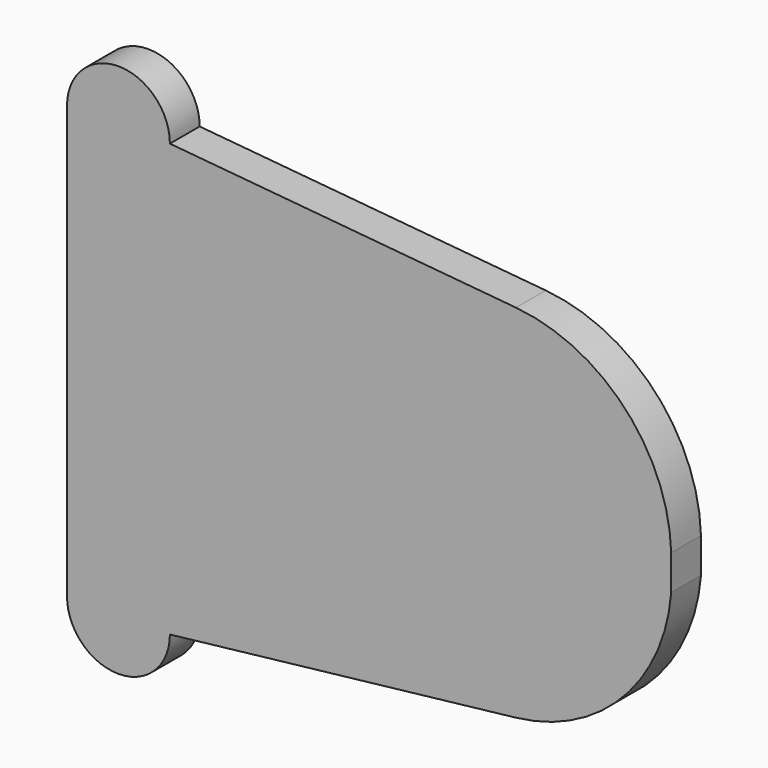
from build123d import *

# Parameters (mm, degrees)
F1_DEPTH = 6.7056


# Not quite as in the source:
# - the program builds the solid bodies; features that only make, move or delete a surface that nothing else refers to are left out


with BuildPart() as f1:
    # F0 (on Front) → F1 (new body)
    with BuildSketch(Plane.XZ):
        with BuildLine():
            ThreePointArc((-32.0095643401, 38.8673432171), (-41.2789452821, 48.1367241591), (-50.5483262241, 38.8673432171))
            Line((-50.5483262241, 38.8673432171), (-50.5483262241, -38.9954559505))
            ThreePointArc((-50.5483262241, -38.9954559505), (-41.2789452821, -48.2648368925), (-32.0095643401, -38.9954559505))
            Line((-32.0095643401, -38.9954559505), (30.3480885923, -31.9170206785))
            ThreePointArc((30.3480885923, -31.9170206785), (49.5331583117, -22.4657405577), (58.3247691393, -2.9695569538))
            Line((58.3247691393, -2.9695569538), (58.3247691393, 3.3366130665))
            ThreePointArc((58.3247691393, 3.3366130665), (49.99023947, 23.5446765042), (30.3480885923, 33.1371799111))
            Line((30.3480885923, 33.1371799111), (-32.0095643401, 38.8673432171))
        make_face()
    extrude(amount=F1_DEPTH)


solid = f1.part
